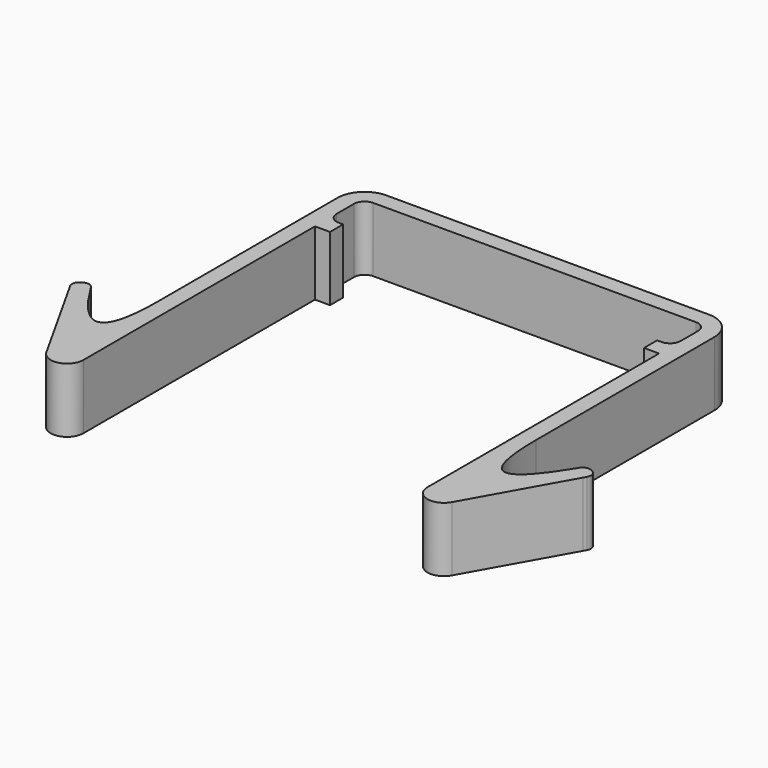
from build123d import *

# Parameters (mm, degrees)
F1_DEPTH    = 15
F2_T1_DEPTH = 15


# Not quite as in the source:
# - a fillet or chamfer that OpenCascade refuses, or shapes differently, is made with other operations: its cross-section is extruded or revolved along the edge and cut away or added


with BuildPart() as f1:
    # F0 (on Top) → F1 (new body)
    with BuildSketch(Plane.XY):
        with BuildLine():
            ThreePointArc((-40, 41.475575803), (-39.267766953, 43.243342756), (-37.5, 43.975575803))
            Line((-37.5, 43.975575803), (0, 43.975575803))
            Line((0, 43.975575803), (0, 47.775575803))
            Line((0, 47.775575803), (-37.5, 47.775575803))
            ThreePointArc((-37.5, 47.775575803), (-41.9618437893, 45.9274195923), (-43.81, 41.465575803))
            Line((-43.81, 41.465575803), (-43.81, 36.475575803))
            Line((-43.81, 36.475575803), (-43.81, -27.529513372))
            Line((-43.81, -27.529513372), (-43.81, -37.104424197))
            Line((-43.81, -37.104424197), (-48.4908909885, -28.7516895034))
            Line((-48.4908909885, -28.7516895034), (-56.369773679, -14.6923540142))
            Line((-56.369773679, -14.6923540142), (-56.7601447269, -13.9957631722))
            ThreePointArc((-56.7601447269, -13.9957631722), (-57.782169231, -13.1905372922), (-59.0742303685, -13.3438370694))
            Line((-59.0742303685, -13.3438370694), (-59.2530634296, -13.4440555122))
            Line((-59.2530634296, -13.4440555122), (-59.4318964906, -13.5442739549))
            ThreePointArc((-59.4318964906, -13.5442739549), (-60.2371223706, -14.566298459), (-60.0838225934, -15.8583595965))
            Line((-60.0838225934, -15.8583595965), (-59.6934515455, -16.5549504386))
            Line((-59.6934515455, -16.5549504386), (-47.1336778665, -38.9670206213))
            ThreePointArc((-47.1336778665, -38.9670206213), (-42.8474805641, -40.7908393032), (-40, -37.104424197))
            Line((-40, -37.104424197), (-40, 30.165575803))
            Line((-40, 30.165575803), (-37.5, 30.165575803))
            Line((-37.5, 30.165575803), (-36.5, 30.165575803))
            Line((-36.5, 30.165575803), (-36.5, 33.975575803))
            Line((-36.5, 33.975575803), (-37.5, 33.975575803))
            ThreePointArc((-37.5, 33.975575803), (-39.267766953, 34.7078088501), (-40, 36.475575803))
            Line((-40, 36.475575803), (-40, 41.475575803))
        make_face()
    extrude(amount=F1_DEPTH)

    # F2: fillet of radius 7 on 1 edges, made by hand

    # F2_s2 → F2_t1 (join)
    with BuildSketch(Plane.XY):
        with BuildLine():
            add(Edge.make_bspline(
                [(-56.7906958843, -13.9434544078), (-43.81, -35.286127782), (-43.81, -10.30597221)],
                knots=[0, 0, 0, 1, 1, 1], degree=2, weights=[1, 1, 1]))
            Line((-43.81, -10.30597221), (-43.11, -10.30597221))
            Line((-43.11, -10.30597221), (-43.11, -37.104424197))
            Line((-43.11, -37.104424197), (-44.4206494768, -37.4466335138))
            ThreePointArc((-44.4206494768, -37.4466335138), (-57.3707942037, -14.337972489), (-57.3887654728, -14.3072026276))
            Line((-57.3887654728, -14.3072026276), (-56.7906958843, -13.9434544078))
        make_face()
    extrude(amount=F2_T1_DEPTH)

    # F3: F1 across face


with BuildPart() as f1_1:
    add(f1.part)
    add(f1.part.mirror(Plane(origin=(0, 45.875575803, 7.5), x_dir=(0, 1, 0), z_dir=(1, 0, 0))))


solid = f1_1.part
